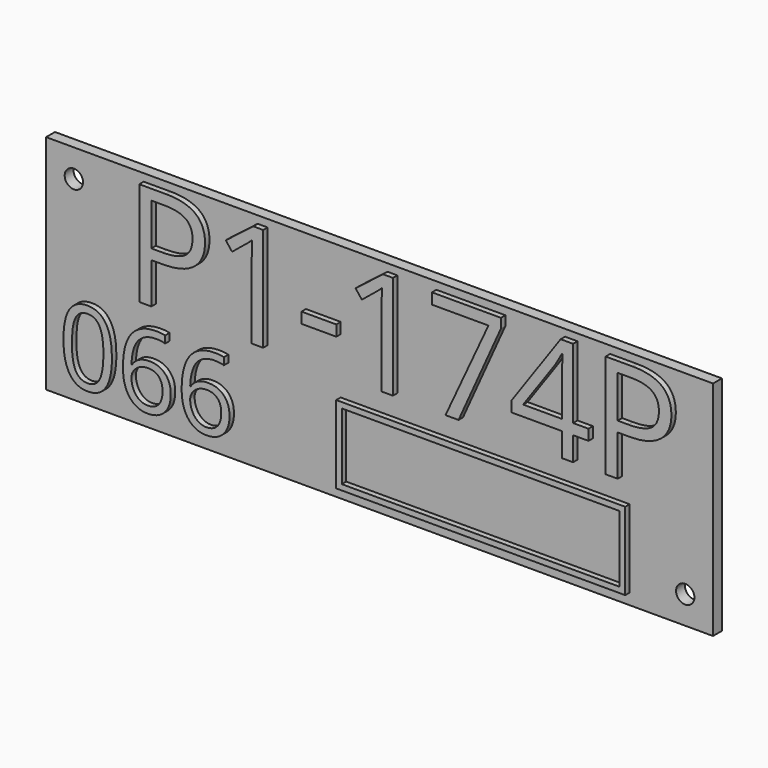
from build123d import *

# Parameters (mm, degrees)
F0_W         = 120
F0_H         = 40
F1_DEPTH     = 2
F3_D         = 3.3
F4_TEXT_SIZE = 26.1352499183
F5_DEPTH     = 1
F6_TEXT_SIZE = 18.4837545126
F7_DEPTH     = 1
F8_W         = 52
F8_H         = 14
F8_W_2       = 49.99999962
F8_H_2       = 11.99999962
F9_DEPTH     = 1


# Not quite as in the source:
# - Text() gives the source's letters only with a copy of the font that has no kerning and outlines rounded to 1/6400 em; it was checked with that copy


with BuildPart() as f1:
    # F0 (on Front) → F1 (new body)
    with BuildSketch(Plane.XZ):
        Rectangle(F0_W, F0_H)
    extrude(amount=F1_DEPTH)

    # F3 (through all)
    with Locations(Plane.XZ.offset(2)):
        with Locations((-55, 15), (55, -15)):
            Hole(F3_D / 2)

    # F4 (on face) → F5 (join)
    with BuildSketch(Plane.XZ.offset(2)):
        with Locations((-45, 0)):
            Text('P1-174P', F4_TEXT_SIZE, font='Open Sans', text_align=(TextAlign.LEFT, TextAlign.BOTTOM))
    extrude(amount=F5_DEPTH)

    # F6 (on face) → F7 (join)
    with BuildSketch(Plane.XZ.offset(2)):
        with Locations((-57, -17)):
            Text('066', F6_TEXT_SIZE, font='Open Sans', text_align=(TextAlign.LEFT, TextAlign.BOTTOM))
    extrude(amount=F7_DEPTH)

    # F8 (on face) → F9 (join)
    with BuildSketch(Plane.XZ.offset(2)):
        with Locations((19, -11)):
            Rectangle(F8_W, F8_H)
        with Locations((19, -11)):
            Rectangle(F8_W_2, F8_H_2, mode=Mode.SUBTRACT)
    extrude(amount=F9_DEPTH)


solid = f1.part
